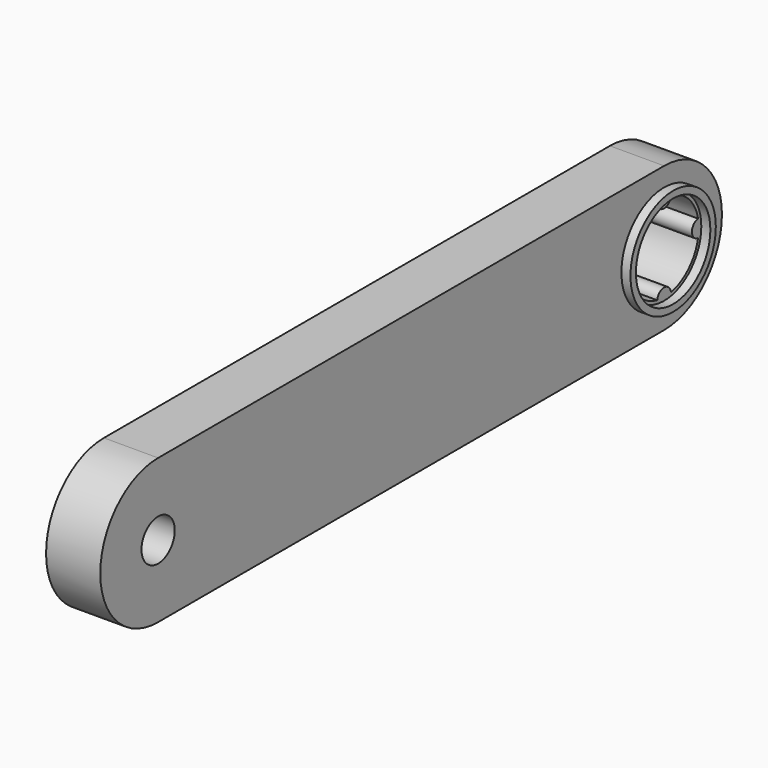
from build123d import *

# Parameters (mm, degrees)
F1_DEPTH = 15
F2_R     = 14.76375
F2_R_2   = 12.875
F3_DEPTH = 2.5
F5_D     = 11.50874


with BuildPart() as f1:
    # F0 (on Right) → F1 (new body)
    with BuildSketch(Plane.YZ):
        with BuildLine():
            Line((-175, -20), (0, -20))
            ThreePointArc((0, -20), (20, 0), (0, 20))
            Line((0, 20), (-175, 20))
            ThreePointArc((-175, 20), (-195, 0), (-175, -20))
        make_face()
        with BuildLine():
            ThreePointArc((-11.7637353516, 2.3695000693), (-8.4852813742, 8.4852813742), (-2.3695000693, 11.7637353516))
            ThreePointArc((-2.3695000693, 11.7637353516), (0, 9.61875), (2.3695000693, 11.7637353516))
            ThreePointArc((2.3695000693, 11.7637353516), (8.4852813742, 8.4852813742), (11.7637353516, 2.3695000693))
            ThreePointArc((11.7637353516, 2.3695000693), (9.61875, 0), (11.7637353516, -2.3695000693))
            ThreePointArc((11.7637353516, -2.3695000693), (8.4852813742, -8.4852813742), (2.3695000693, -11.7637353516))
            ThreePointArc((2.3695000693, -11.7637353516), (0, -9.61875), (-2.3695000693, -11.7637353516))
            ThreePointArc((-2.3695000693, -11.7637353516), (-8.4852813742, -8.4852813742), (-11.7637353516, -2.3695000693))
            ThreePointArc((-11.7637353516, -2.3695000693), (-9.61875, 0), (-11.7637353516, 2.3695000693))
        make_face(mode=Mode.SUBTRACT)
    extrude(amount=F1_DEPTH)

    # F2 (on face) → F3 (join)
    with BuildSketch(Plane.YZ.offset(15)):
        Circle(F2_R)
        Circle(F2_R_2, mode=Mode.SUBTRACT)
    extrude(amount=F3_DEPTH)

    # F5 (through all)
    with Locations(Plane.YZ.offset(15)):
        with Locations((-175, 0)):
            Hole(F5_D / 2)


solid = f1.part
